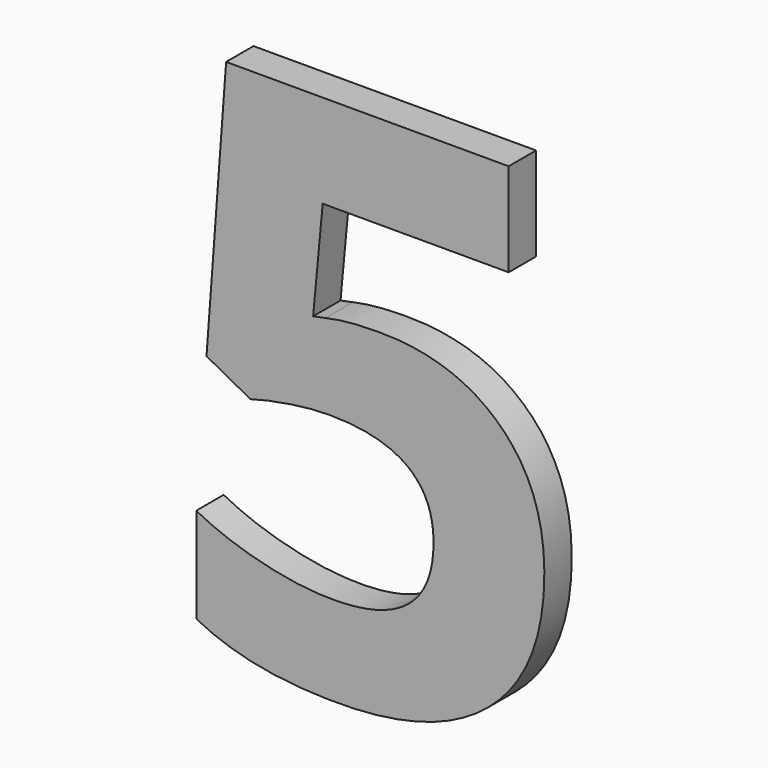
from build123d import *

# Parameters (mm, degrees)
F0_TEXT_SIZE = 85.235066298
F1_DEPTH     = 4


# Not quite as in the source:
# - Text() gives the source's letters only with a copy of the font that has no kerning and outlines rounded to 1/6400 em; it was checked with that copy


with BuildPart() as f1:
    # F0 (on Front) → F1 (new body)
    with BuildSketch(Plane.XZ):
        with Locations((0, 0)):
            Text('5', F0_TEXT_SIZE, font='Open Sans', font_style=FontStyle.BOLD, text_align=(TextAlign.LEFT, TextAlign.BOTTOM))
    extrude(amount=F1_DEPTH)


solid = f1.part
